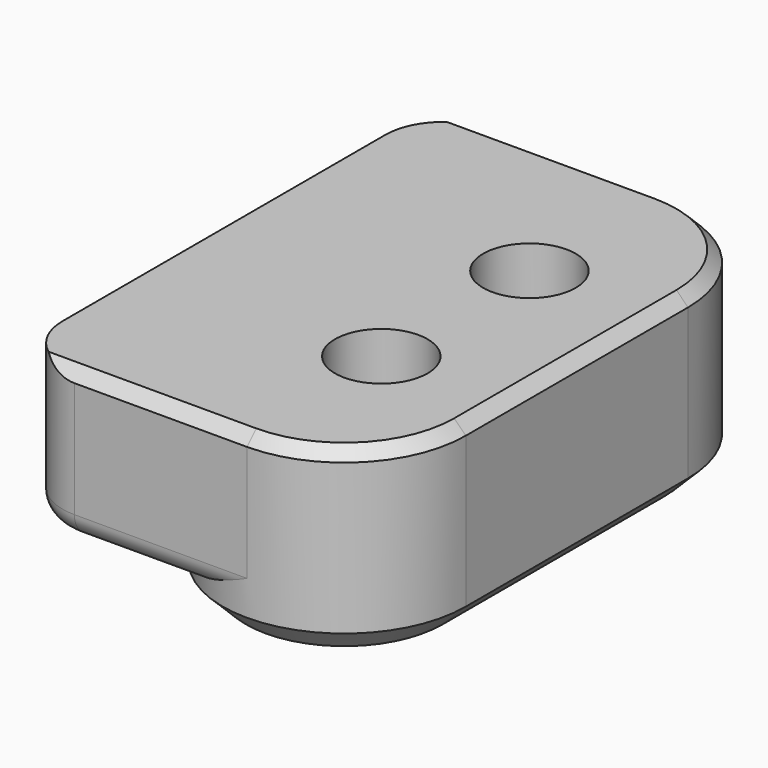
from build123d import *

# Parameters (mm, degrees)
F0_R         = 2
F1_DEPTH     = 1.5
F2_R         = 2
F3_DEPTH     = 6.5
F4_SIZE      = 1
F5_T1_DEPTH  = 27.5
F5_T6_DEPTH  = 16.75
F5_S7_R      = 5.25
F5_T8_DEPTH  = 10
F5_T12_DEPTH = 16.75
F5_S13_R     = 5.25
F5_T14_DEPTH = 10
F6_SIZE      = 0.5
F7_R         = 0.5
F8_T1_DEPTH  = 12.35
F8_T4_ANGLE  = 90
F8_T6_ANGLE  = 90


# Not quite as in the source:
# - a fillet or chamfer that OpenCascade refuses, or shapes differently, is made with other operations: its cross-section is extruded or revolved along the edge and cut away or added


with BuildPart() as f1:
    # F0 (on Top) → F1 (new body)
    with BuildSketch(Plane.XY):
        with BuildLine():
            ThreePointArc((38.3721691668, 6.4511308521), (33.1221691668, 11.7011308521), (27.8721691668, 6.4511308521))
            Line((27.8721691668, 6.4511308521), (27.8721691668, -5.5488691479))
            ThreePointArc((27.8721691668, -5.5488691479), (33.1221691668, -10.7988691479), (38.3721691668, -5.5488691479))
            Line((38.3721691668, -5.5488691479), (38.3721691668, 6.4511308521))
        make_face()
        with Locations((33.1221691668, -3.5488691479)):
            Circle(F0_R, mode=Mode.SUBTRACT)
        with Locations((33.1221691668, 4.4511308521)):
            Circle(F0_R, mode=Mode.SUBTRACT)
    extrude(amount=F1_DEPTH)

    # F2 (on face) → F3 (join)
    with BuildSketch(Plane.XY.offset(1.5)):
        with BuildLine():
            Line((38.3721691668, -5.5488691479), (38.3721691668, 6.4511308521))
            ThreePointArc((38.3721691668, 6.4511308521), (36.834479768, 10.1634414533), (33.1221691668, 11.7011308521))
            Line((33.1221691668, 11.7011308521), (23.1221691668, 11.7011308521))
            Line((23.1221691668, 11.7011308521), (23.1221691668, -10.7988691479))
            Line((23.1221691668, -10.7988691479), (33.1221691668, -10.7988691479))
            ThreePointArc((33.1221691668, -10.7988691479), (36.834479768, -9.2611797491), (38.3721691668, -5.5488691479))
        make_face()
        with Locations((33.1221691668, -3.5488691479)):
            Circle(F2_R, mode=Mode.SUBTRACT)
        with Locations((33.1221691668, 4.4511308521)):
            Circle(F2_R, mode=Mode.SUBTRACT)
    extrude(amount=F3_DEPTH)

    # F4
    f4_edges = [f1.edges().sort_by_distance(p)[0] for p in [
        (27.872169, 0.451131, 0),
        (38.372169, 0.451131, 0),
        (33.122169, 11.701131, 0),
        (33.122169, -10.798869, 0),
    ]]
    chamfer(f4_edges, length=F4_SIZE)

    # F5: fillet of radius 1 on 3 edges, made by hand

    # F5_s2 → F5_t1 (cut)
    with BuildSketch(Plane.XZ.offset(-14.2011308521)):
        with BuildLine():
            ThreePointArc((24.1221691668, 1.5), (23.4150623856, 1.7928932188), (23.1221691668, 2.5))
            Line((23.1221691668, 2.5), (23.1221691668, 1.5))
            Line((23.1221691668, 1.5), (24.1221691668, 1.5))
        make_face()
    extrude(amount=F5_T1_DEPTH, mode=Mode.SUBTRACT)


with BuildPart() as f5_tool4:
    # F5_s5 → F5_t6 (new body)
    with BuildSketch(Plane.YZ.offset(37.3721691668)):
        with BuildLine():
            ThreePointArc((10.7011308521, 1.5), (11.4082376333, 1.7928932188), (11.7011308521, 2.5))
            Line((11.7011308521, 2.5), (11.7011308521, 1.5))
            Line((11.7011308521, 1.5), (10.7011308521, 1.5))
        make_face()
    extrude(amount=-F5_T6_DEPTH)

    # F5_s7 → F5_t8 (cut, symmetric)
    with BuildSketch(Plane.XY.offset(2)):
        with Locations((33.1221691668, 6.4511308521)):
            Circle(F5_S7_R)
    extrude(amount=F5_T8_DEPTH, both=True, mode=Mode.SUBTRACT)


with BuildPart() as f1_1:
    add(f1.part)

    # F5_t3: cut F5_tool4
    add(f5_tool4.part, mode=Mode.SUBTRACT)


with BuildPart() as f5_tool10:
    # F5_s11 → F5_t12 (new body)
    with BuildSketch(Plane.YZ.offset(20.6221691668)):
        with BuildLine():
            ThreePointArc((-9.7988691479, 1.5), (-10.5059759291, 1.7928932188), (-10.7988691479, 2.5))
            Line((-10.7988691479, 2.5), (-10.7988691479, 1.5))
            Line((-10.7988691479, 1.5), (-9.7988691479, 1.5))
        make_face()
    extrude(amount=F5_T12_DEPTH)

    # F5_s13 → F5_t14 (cut, symmetric)
    with BuildSketch(Plane.XY.offset(2)):
        with Locations((33.1221691668, -5.5488691479)):
            Circle(F5_S13_R)
    extrude(amount=F5_T14_DEPTH, both=True, mode=Mode.SUBTRACT)


with BuildPart() as f1_2:
    add(f1_1.part)

    # F5_t9: cut F5_tool10
    add(f5_tool10.part, mode=Mode.SUBTRACT)

    # F6
    f6_edges = [f1_2.edges().sort_by_distance(p)[0] for p in [
        (28.122169, 11.701131, 8),
        (38.372169, 0.451131, 8),
        (36.83448, -9.26118, 8),
        (36.83448, 10.163441, 8),
        (28.122169, -10.798869, 8),
    ]]
    chamfer(f6_edges, length=F6_SIZE)

    # F7
    f7_edges = [f1_2.edges().sort_by_distance(p)[0] for p in [
        (31.122169, -3.548869, 0),
        (31.122169, 4.451131, 0),
    ]]
    fillet(f7_edges, radius=F7_R)

    # F8: fillet of radius 2.54 on 2 edges, made by hand

    # F8_s2 → F8_t1 (cut)
    with BuildSketch(Plane.XY.offset(1.5)):
        with BuildLine():
            ThreePointArc((25.6621691668, 11.7011308521), (23.8661179426, 10.9571820763), (23.1221691668, 9.1611308521))
            Line((23.1221691668, 9.1611308521), (23.1221691668, 11.7011308521))
            Line((23.1221691668, 11.7011308521), (25.6621691668, 11.7011308521))
        make_face()
        with BuildLine():
            ThreePointArc((25.6621691668, -10.7988691479), (23.8661179426, -10.0549203721), (23.1221691668, -8.2588691479))
            Line((23.1221691668, -8.2588691479), (23.1221691668, -10.7988691479))
            Line((23.1221691668, -10.7988691479), (25.6621691668, -10.7988691479))
        make_face()
    extrude(amount=F8_T1_DEPTH, mode=Mode.SUBTRACT)

    # F8_s3 → F8_t4 (revolve, cut)
    with BuildSketch(Plane.YZ.offset(25.6621691668)):
        with BuildLine():
            ThreePointArc((-9.7988691479, 1.5), (-10.5059759291, 1.7928932188), (-10.7988691479, 2.5))
            Line((-10.7988691479, 2.5), (-10.7988691479, 1.5))
            Line((-10.7988691479, 1.5), (-9.7988691479, 1.5))
        make_face()
    revolve(axis=Axis((25.6621691668, -8.2588691479, 1.5), (0, 0, -1)), revolution_arc=F8_T4_ANGLE, mode=Mode.SUBTRACT)

    # F8_s5 → F8_t6 (revolve, cut)
    with BuildSketch(Plane.XZ.offset(-9.1611308521)):
        with BuildLine():
            ThreePointArc((24.1221691668, 1.5), (23.4150623856, 1.7928932188), (23.1221691668, 2.5))
            Line((23.1221691668, 2.5), (23.1221691668, 1.5))
            Line((23.1221691668, 1.5), (24.1221691668, 1.5))
        make_face()
    revolve(axis=Axis((25.6621691668, 9.1611308521, 1.5), (0, 0, -1)), revolution_arc=F8_T6_ANGLE, mode=Mode.SUBTRACT)


solid = f1_2.part
